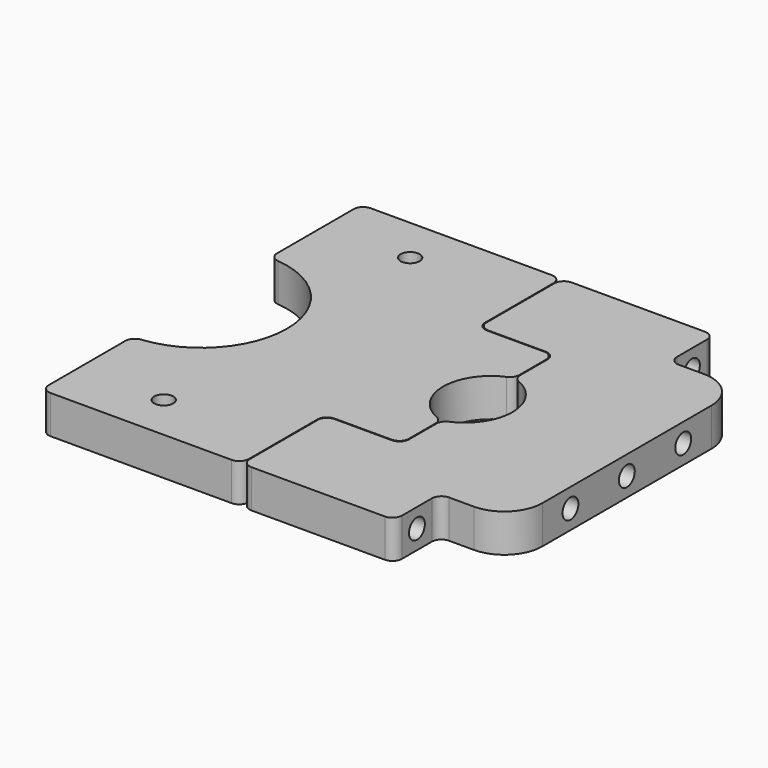
from build123d import *

# Parameters (mm, degrees)
F0_R      = 6.35
F1_DEPTH  = 47.625
F3_DEPTH  = 31.75
F4_R      = 23.8125
F4_R_2    = 18.7325
F5_DEPTH  = 20.32
F6_R      = 6.35
F6_R_2    = 2.2225
F7_DEPTH  = 14.605
F8_R      = 54.5973
F8_R_2    = 6.35
F9_DEPTH  = 118.491
F10_R     = 54.61
F10_R_2   = 54.5973
F10_R_3   = 6.35
F11_DEPTH = 57.15
F13_DEPTH = 101.6
F15_DEPTH = 25.4
F16_DEPTH = 76.2
F18_DEPTH = 76.2
F20_D     = 12.7
F20_DEPTH = 12.7
F20_TIP   = 3.8154649308
F22_D     = 12.7
F22_2_D   = 12.7
F23_R     = 5.08
F23_2_R   = 5.08
F26_R     = 6.35
F27_R     = 3.175
F28_DEPTH = 12.7
F33_DEPTH = 12.7
F34_R     = 3.175
F35_R     = 3.175
F36_R     = 12.7
F38_D     = 6.604
F38_DEPTH = 50.8
F38_TIP   = 1.984041764
F40_D     = 6.604
F40_DEPTH = 50.8
F40_TIP   = 1.984041764
F42_D     = 6.604
F42_DEPTH = 50.8
F42_TIP   = 1.984041764
F44_D     = 5.1054
F44_DEPTH = 25.4
F44_TIP   = 1.5338169022
F46_D     = 5.1054
F46_DEPTH = 25.4
F46_TIP   = 1.5338169022
F48_D     = 5.1054
F48_DEPTH = 25.4
F48_TIP   = 1.5338169022


# Not quite as in the source:
# - a feature names something its author has since deleted; it is built from what else it names


with BuildPart() as f1:
    # F0 (on Top) → F1 (new body)
    with BuildSketch(Plane.XY):
        Circle(F0_R)
    extrude(amount=-F1_DEPTH)

    # F2 (on face) → F3 (cut)
    with BuildSketch(Plane.XY):
        with BuildLine():
            Line((-3.4925, 5.3032955556), (3.4925, 5.3032955556))
            ThreePointArc((3.4925, 5.3032955556), (0, 6.35), (-3.4925, 5.3032955556))
        make_face()
    extrude(amount=-F3_DEPTH, mode=Mode.SUBTRACT)


with BuildPart() as f5:
    # F4 (on face) → F5 (new body)
    with BuildSketch(Plane(origin=(0, 0, -47.625), x_dir=(1, 0, 0), z_dir=(0, 0, -1))):
        Circle(F4_R)
        Circle(F4_R_2, mode=Mode.SUBTRACT)
    extrude(amount=-F5_DEPTH)


with BuildPart() as f7:
    # F6 (on face) → F7 (new body)
    with BuildSketch(Plane(origin=(0, 0, -47.625), x_dir=(1, 0, 0), z_dir=(0, 0, -1))):
        with BuildLine():
            ThreePointArc((30.5321277528, -45.2773814933), (48.216239985, -25.640715702), (54.61, 0))
            ThreePointArc((54.61, 0), (48.216239985, 25.640715702), (30.5321277528, 45.2773814933))
            ThreePointArc((30.5321277528, 45.2773814933), (26.567027027, 47.7121072155), (22.4090607059, 49.800462832))
            ThreePointArc((22.4090607059, 49.800462832), (0, 54.61), (-22.4090607059, 49.800462832))
            ThreePointArc((-22.4090607059, 49.800462832), (-26.567027027, 47.7121072155), (-30.5321277528, 45.2773814933))
            ThreePointArc((-30.5321277528, 45.2773814933), (-54.61, 0), (-30.5321277528, -45.2773814933))
            ThreePointArc((-30.5321277528, -45.2773814933), (-26.567027027, -47.7121072155), (-22.4090607059, -49.800462832))
            ThreePointArc((-22.4090607059, -49.800462832), (0, -54.61), (22.4090607059, -49.800462832))
            ThreePointArc((22.4090607059, -49.800462832), (26.567027027, -47.7121072155), (30.5321277528, -45.2773814933))
        make_face()
        Circle(F6_R, mode=Mode.SUBTRACT)
        with BuildLine():
            ThreePointArc((-30.5321277528, -45.2773814933), (-31.6641891892, -56.8661742976), (-22.4090607059, -49.800462832))
            ThreePointArc((-22.4090607059, -49.800462832), (-26.567027027, -47.7121072155), (-30.5321277528, -45.2773814933))
        make_face()
        with Locations((-28.575, -51.3182548539)):
            Circle(F6_R_2, mode=Mode.SUBTRACT)
        with BuildLine():
            ThreePointArc((22.4090607059, -49.800462832), (31.6641891892, -56.8661742976), (30.5321277528, -45.2773814933))
            ThreePointArc((30.5321277528, -45.2773814933), (26.567027027, -47.7121072155), (22.4090607059, -49.800462832))
        make_face()
        with Locations((28.575, -51.3182548539)):
            Circle(F6_R_2, mode=Mode.SUBTRACT)
        with BuildLine():
            ThreePointArc((22.4090607059, 49.800462832), (26.567027027, 47.7121072155), (30.5321277528, 45.2773814933))
            ThreePointArc((30.5321277528, 45.2773814933), (31.6641891892, 56.8661742976), (22.4090607059, 49.800462832))
        make_face()
        with Locations((28.575, 51.3182548539)):
            Circle(F6_R_2, mode=Mode.SUBTRACT)
        with BuildLine():
            ThreePointArc((-30.5321277528, 45.2773814933), (-26.567027027, 47.7121072155), (-22.4090607059, 49.800462832))
            ThreePointArc((-22.4090607059, 49.800462832), (-31.6641891892, 56.8661742976), (-30.5321277528, 45.2773814933))
        make_face()
        with Locations((-28.575, 51.3182548539)):
            Circle(F6_R_2, mode=Mode.SUBTRACT)
    extrude(amount=F7_DEPTH)

    # F8 (on face) → F9 (join)
    with BuildSketch(Plane(origin=(0, 0, -62.23), x_dir=(1, 0, 0), z_dir=(0, 0, -1))):
        Circle(F8_R)
        Circle(F8_R_2, mode=Mode.SUBTRACT)
    extrude(amount=F9_DEPTH)

    # F10 (on face) → F11 (join)
    with BuildSketch(Plane(origin=(0, 0, -180.721), x_dir=(1, 0, 0), z_dir=(0, 0, -1))):
        Circle(F10_R)
        Circle(F10_R_2, mode=Mode.SUBTRACT)
        Circle(F10_R_2)
        Circle(F10_R_3, mode=Mode.SUBTRACT)
    extrude(amount=F11_DEPTH)

    # F26
    f26_edges = [f7.edges().sort_by_distance(p)[0] for p in [
        (-22.409061, -49.800463, -54.9275),
        (30.532128, -45.277381, -54.9275),
        (22.409061, 49.800463, -54.9275),
        (-30.532128, 45.277381, -54.9275),
    ]]
    fillet(f26_edges, radius=F26_R)


with BuildPart() as f13:
    # F12 (on face) → F13 (new body)
    with BuildSketch(Plane.XY.offset(-47.625)):
        with BuildLine():
            Line((-82.55, 31.7245898319), (-44.45, 31.7245898319))
            ThreePointArc((-44.45, 31.7245898319), (-38.0985486737, 39.1248346829), (-30.5321277528, 45.2773814933))
            ThreePointArc((-30.5321277528, 45.2773814933), (-31.6641891892, 56.8661742976), (-22.4090607059, 49.800462832))
            ThreePointArc((-22.4090607059, 49.800462832), (-11.4596863994, 53.3940791439), (0, 54.61))
            Line((0, 54.61), (0, 67.31))
            ThreePointArc((0, 67.31), (-26.9947671741, 61.30558596), (-48.8991597124, 44.4245898319))
            Line((-48.8991597124, 44.4245898319), (-82.55, 44.4245898319))
            Line((-82.55, 44.4245898319), (-82.55, 31.7245898319))
        make_face()
        with BuildLine():
            ThreePointArc((30.5321277528, 45.2773814933), (38.0985486737, 39.1248346829), (44.45, 31.7245898319))
            Line((44.45, 31.7245898319), (82.55, 31.7245898319))
            Line((82.55, 31.7245898319), (82.55, 44.4245898319))
            Line((82.55, 44.4245898319), (48.8991597124, 44.4245898319))
            ThreePointArc((48.8991597124, 44.4245898319), (26.9947671741, 61.30558596), (0, 67.31))
            Line((0, 67.31), (0, 54.61))
            ThreePointArc((0, 54.61), (11.4596863994, 53.3940791439), (22.4090607059, 49.800462832))
            ThreePointArc((22.4090607059, 49.800462832), (31.6641891892, 56.8661742976), (30.5321277528, 45.2773814933))
        make_face()
    extrude(amount=-F13_DEPTH)

    # F22 (through all)
    with Locations(Plane.XZ.offset(44.4245898319)):
        with Locations((-69.85, -60.325), (-69.85, -98.425), (-69.85, -136.525), (69.85, -60.325), (69.85, -98.425), (69.85, -136.525)):
            Hole(F22_D / 2)

    # F23
    f23_edges = [f13.edges().sort_by_distance(p)[0] for p in [
        (-48.89916, 44.42459, -98.425),
        (48.89916, 44.42459, -98.425),
    ]]
    fillet(f23_edges, radius=F23_R)


with BuildPart() as f15:
    # F14 (on face) → F15 (new body)
    with BuildSketch(Plane.XY.offset(-47.625)):
        with BuildLine():
            Line((82.55, -31.7245898319), (44.45, -31.7245898319))
            ThreePointArc((44.45, -31.7245898319), (38.0985486737, -39.1248346829), (30.5321277528, -45.2773814933))
            ThreePointArc((30.5321277528, -45.2773814933), (31.6641891892, -56.8661742976), (22.4090607059, -49.800462832))
            ThreePointArc((22.4090607059, -49.800462832), (11.4596863994, -53.3940791439), (0, -54.61))
            Line((0, -54.61), (0, -67.31))
            ThreePointArc((0, -67.31), (26.9947671741, -61.30558596), (48.8991597124, -44.4245898319))
            Line((48.8991597124, -44.4245898319), (82.55, -44.4245898319))
            Line((82.55, -44.4245898319), (82.55, -31.7245898319))
        make_face()
        with BuildLine():
            ThreePointArc((-30.5321277528, -45.2773814933), (-38.0985486737, -39.1248346829), (-44.45, -31.7245898319))
            Line((-44.45, -31.7245898319), (-82.55, -31.7245898319))
            Line((-82.55, -31.7245898319), (-82.55, -44.4245898319))
            Line((-82.55, -44.4245898319), (-48.8991597124, -44.4245898319))
            ThreePointArc((-48.8991597124, -44.4245898319), (-26.9947671741, -61.30558596), (0, -67.31))
            Line((0, -67.31), (0, -54.61))
            ThreePointArc((0, -54.61), (-11.4596863994, -53.3940791439), (-22.4090607059, -49.800462832))
            ThreePointArc((-22.4090607059, -49.800462832), (-31.6641891892, -56.8661742976), (-30.5321277528, -45.2773814933))
        make_face()
    extrude(amount=-F15_DEPTH)

    # F16 (add): faces of the model
    f16_faces = [f15.faces().sort_by_distance(p)[0] for p in [
        (80.8610852178, -38.0745898319, -73.025),
        (80.8610852178, -38.0745898319, -73.025),
    ]]
    extrude(f16_faces, amount=F16_DEPTH)

    # F17 (on face) → F18 (join)
    with BuildSketch(Plane(origin=(0, 0, -149.225), x_dir=(1, 0, 0), z_dir=(0, 0, -1))):
        with BuildLine():
            Line((-38.1, 87.6758182624), (-38.1, 54.6558182624))
            ThreePointArc((-38.1, 54.6558182624), (0, 67.31), (38.1, 54.6558182624))
            Line((38.1, 54.6558182624), (38.1, 87.6758182624))
            Line((38.1, 87.6758182624), (12.7, 87.6758182624))
            ThreePointArc((12.7, 87.6758182624), (0, 76.2), (-12.7, 87.6758182624))
            Line((-12.7, 87.6758182624), (-38.1, 87.6758182624))
        make_face()
    extrude(amount=-F18_DEPTH)

    # F20
    with Locations(Plane.XZ.offset(87.6758182624)):
        with Locations((-25.4, -85.725), (25.1709398942, -85.725), (-25.4, -111.125), (24.5334483168, -111.125), (-25.4, -136.525), (25.347779546, -136.525)):
            Hole(F20_D / 2, depth=F20_DEPTH)
            with Locations((0, 0, -(F20_DEPTH + F20_TIP / 2))):  # 118° drill point
                Cone(0, F20_D / 2, F20_TIP, mode=Mode.SUBTRACT)

    # F22#2 (through all)
    with Locations(Plane.XZ.offset(44.4245898319)):
        with Locations((-69.85, -60.325), (-69.85, -98.425), (-69.85, -136.525), (69.85, -60.325), (69.85, -98.425), (69.85, -136.525)):
            Hole(F22_2_D / 2)

    # F23#2
    f23_2_edges = [f15.edges().sort_by_distance(p)[0] for p in [
        (-38.1, -54.655818, -111.125),
        (0, -67.31, -73.025),
        (38.1, -54.655818, -111.125),
        (48.89916, -44.42459, -98.425),
        (-48.89916, -44.42459, -98.425),
    ]]
    fillet(f23_2_edges, radius=F23_2_R)


with BuildPart() as f28:
    # F27 (on Top) → F28 (new body)
    with BuildSketch(Plane.XY):
        with BuildLine():
            ThreePointArc((0, 28.575), (28.575, 0), (0, -28.575))
            Line((0, -28.575), (0, -66.675))
            Line((0, -66.675), (66.675, -66.675))
            Line((66.675, -66.675), (66.675, -31.75))
            Line((66.675, -31.75), (92.075, -31.75))
            Line((92.075, -31.75), (92.075, -15.24))
            ThreePointArc((92.075, -15.24), (80.645, 0), (92.075, 15.24))
            Line((92.075, 15.24), (92.075, 31.75))
            Line((92.075, 31.75), (66.675, 31.75))
            Line((66.675, 31.75), (66.675, 66.675))
            Line((66.675, 66.675), (0, 66.675))
            Line((0, 66.675), (0, 28.575))
        make_face()
        with Locations((28.575, -51.3182548539)):
            Circle(F27_R, mode=Mode.SUBTRACT)
        with Locations((28.575, 51.3182548539)):
            Circle(F27_R, mode=Mode.SUBTRACT)
    extrude(amount=F28_DEPTH)

    # F34
    f34_edges = [f28.edges().sort_by_distance(p)[0] for p in [
        (92.075, -31.75, 6.35),
        (66.675, -31.75, 6.35),
        (66.675, -66.675, 6.35),
        (92.075, -15.24, 6.35),
        (92.075, 15.24, 6.35),
        (92.075, 31.75, 6.35),
        (66.675, 31.75, 6.35),
        (66.675, 66.675, 6.35),
        (0, -66.675, 6.35),
        (0, -28.575, 6.35),
        (0, 28.575, 6.35),
        (0, 66.675, 6.35),
    ]]
    fillet(f34_edges, radius=F34_R)

    # F44
    with Locations(Plane.YZ.offset(66.675)):
        with Locations((-57.277, 6.35)):
            Hole(F44_D / 2, depth=F44_DEPTH)
            with Locations((0, 0, -(F44_DEPTH + F44_TIP / 2))):  # 118° drill point
                Cone(0, F44_D / 2, F44_TIP, mode=Mode.SUBTRACT)

    # F46
    with Locations(Plane.YZ.offset(66.675)):
        with Locations((57.277, 6.35)):
            Hole(F46_D / 2, depth=F46_DEPTH)
            with Locations((0, 0, -(F46_DEPTH + F46_TIP / 2))):  # 118° drill point
                Cone(0, F46_D / 2, F46_TIP, mode=Mode.SUBTRACT)

    # F48
    with Locations(Plane.YZ.offset(92.075)):
        with Locations((-23.495, 6.35), (23.495, 6.35)):
            Hole(F48_D / 2, depth=F48_DEPTH)
            with Locations((0, 0, -(F48_DEPTH + F48_TIP / 2))):  # 118° drill point
                Cone(0, F48_D / 2, F48_TIP, mode=Mode.SUBTRACT)


with BuildPart() as f33:
    # F32 (on face) → F33 (new body)
    with BuildSketch(Plane.XY.offset(12.7)):
        with BuildLine():
            Line((66.929, -32.004), (66.929, -66.675))
            Line((66.929, -66.675), (117.729, -66.675))
            Line((117.729, -66.675), (117.729, -47.879))
            Line((117.729, -47.879), (141.859, -47.879))
            Line((141.859, -47.879), (141.859, 0))
            Line((141.859, 0), (141.859, 47.879))
            Line((141.859, 47.879), (117.729, 47.879))
            Line((117.729, 47.879), (117.729, 66.675))
            Line((117.729, 66.675), (66.929, 66.675))
            Line((66.929, 66.675), (66.929, 32.004))
            Line((66.929, 32.004), (92.329, 32.004))
            Line((92.329, 32.004), (92.329, 15.24))
            ThreePointArc((92.329, 15.24), (103.759, 0), (92.329, -15.24))
            Line((92.329, -15.24), (92.329, -32.004))
            Line((92.329, -32.004), (66.929, -32.004))
        make_face()
    extrude(amount=-F33_DEPTH)

    # F35
    f35_edges = [f33.edges().sort_by_distance(p)[0] for p in [
        (66.929, 32.004, 6.35),
        (92.329, 32.004, 6.35),
        (92.329, 15.24, 6.35),
        (92.329, -15.24, 6.35),
        (92.329, -32.004, 6.35),
        (66.929, -32.004, 6.35),
        (117.729, -66.675, 6.35),
        (117.729, -47.879, 6.35),
        (117.729, 66.675, 6.35),
        (117.729, 47.879, 6.35),
        (66.929, -66.675, 6.35),
        (66.929, 66.675, 6.35),
    ]]
    fillet(f35_edges, radius=F35_R)

    # F36
    f36_edges = [f33.edges().sort_by_distance(p)[0] for p in [
        (141.859, 47.879, 6.35),
        (141.859, -47.879, 6.35),
    ]]
    fillet(f36_edges, radius=F36_R)

    # F38
    with Locations(Plane.YZ.offset(117.729)):
        with Locations((-57.277, 6.35)):
            Hole(F38_D / 2, depth=F38_DEPTH)
            with Locations((0, 0, -(F38_DEPTH + F38_TIP / 2))):  # 118° drill point
                Cone(0, F38_D / 2, F38_TIP, mode=Mode.SUBTRACT)

    # F40
    with Locations(Plane.YZ.offset(117.729)):
        with Locations((57.277, 6.35)):
            Hole(F40_D / 2, depth=F40_DEPTH)
            with Locations((0, 0, -(F40_DEPTH + F40_TIP / 2))):  # 118° drill point
                Cone(0, F40_D / 2, F40_TIP, mode=Mode.SUBTRACT)

    # F42
    with Locations(Plane.YZ.offset(141.859)):
        with Locations((-23.495, 6.35), (23.495, 6.35), (0, 6.35)):
            Hole(F42_D / 2, depth=F42_DEPTH)
            with Locations((0, 0, -(F42_DEPTH + F42_TIP / 2))):  # 118° drill point
                Cone(0, F42_D / 2, F42_TIP, mode=Mode.SUBTRACT)


solid = Compound([f28.part, f33.part])
